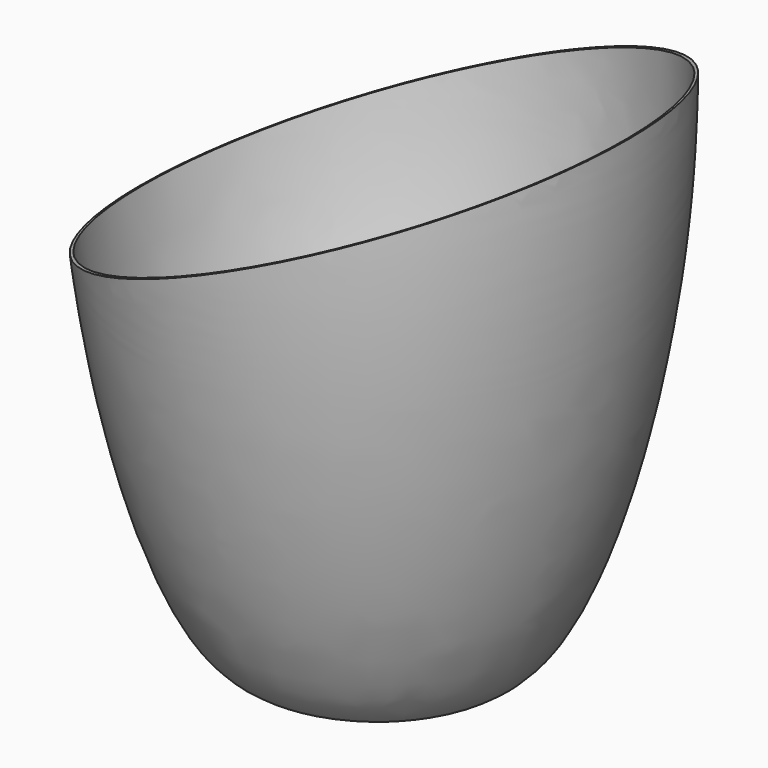
from build123d import *

# Parameters (mm, degrees)
F3_DEPTH      = 87.2
F3_DEPTH_BACK = 108.3


# Not quite as in the source:
# - the dataset's text gives a spline's control points without its knots; the knots are read off the source's solid


with BuildPart() as f1:
    # F0 (on Front) → F1 (revolve)
    with BuildSketch(Plane.XZ):
        with BuildLine():
            Line((-26, 0), (-24, 0))
            Line((-24, 0), (-24, 0.7))
            Line((-24, 0.7), (-26.000231048, 0.6999925375))
            add(Edge.make_bspline(
                [(-26.000231048, 0.6999925375), (-42.4469747777, 0.7759363516), (-61.0256584264, 71.094551837), (-60, 130)],
                knots=[0, 0, 0, 0, 133.6954607255, 133.6954607255, 133.6954607255, 133.6954607255], degree=3))
            Line((-60, 130), (-60.6998939126, 130.0121865143))
            add(Edge.make_bspline(
                [(-26.0034633051, 0), (-26.5796975271, 0.0026607957), (-27.7321648969, 0.1624599653), (-29.4295260176, 0.8298855591), (-31.0900677324, 1.8863905392), (-32.7200814566, 3.3051792178), (-34.3256546626, 5.0676867813), (-36.4380461904, 7.8560362741), (-39.0277431424, 12.1288455713), (-42.0418595357, 18.4061797237), (-44.9382391494, 25.72048285), (-47.6888169613, 33.9561861991), (-50.2636113567, 42.996233753), (-52.631812031, 52.7227009583), (-55.4722689862, 66.4486378575), (-58.3495045205, 84.7292737665), (-60.4712587342, 107.5117720052), (-60.8284425216, 122.6294036772), (-60.6998939126, 130.0121865143)],
                knots=[0, 0, 0, 0, 0.03125, 0.0625, 0.09375, 0.125, 0.15625, 0.1875, 0.25, 0.3125, 0.375, 0.4375, 0.5, 0.5625, 0.625, 0.75, 0.875, 1, 1, 1, 1], degree=3))
            Line((-26.0034633051, 0), (-26, 0))
        make_face()
    revolve(axis=Axis((0, 0, 39.7031084829), (0, 0, 1)))

    # F2 (on Front) → F3 (cut, two sides)
    with BuildSketch(Plane.XZ) as f3_sk:
        Polygon((-75.4877477884, 74.1103456458), (66.8336823583, 132.2212533196), (66.8336823583, 154.84363), (-75.4877477884, 154.84363), align=None)
    extrude(amount=-F3_DEPTH, mode=Mode.SUBTRACT)
    extrude(f3_sk.sketch, amount=F3_DEPTH_BACK, mode=Mode.SUBTRACT)


solid = f1.part
